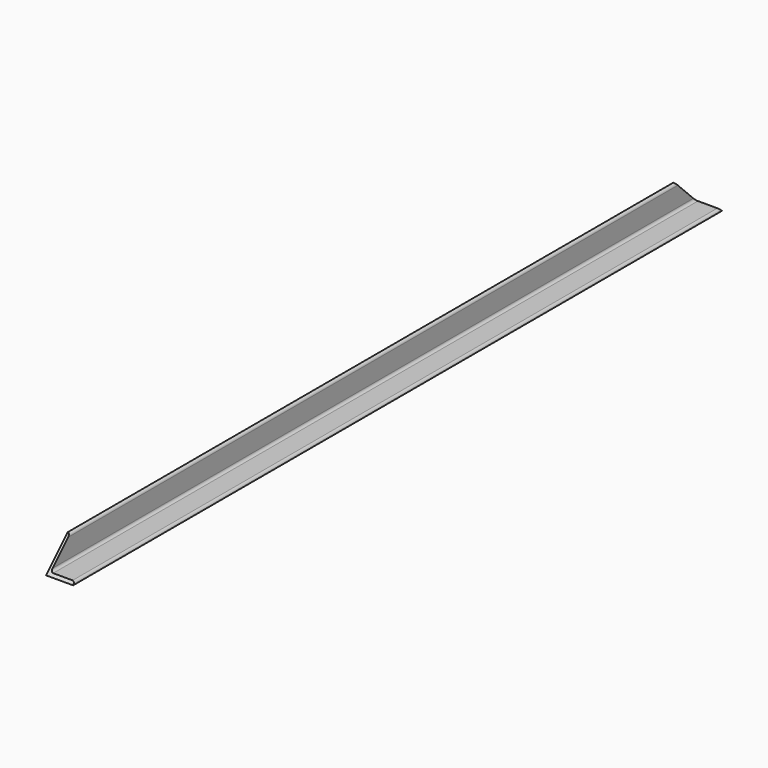
from build123d import *

# Parameters (mm, degrees)
F2_DEPTH = 1524
F4_DEPTH = 50.8


# Not quite as in the source:
# - a variable given as a bare number and used for a length is read in inches; the dataset says mm whatever the document's units were


with BuildPart() as f2:
    # F1 (on Front) → F2 (new body)
    with BuildSketch(Plane.XZ):
        with BuildLine():
            ThreePointArc((4.7625, -4.7625), (3.3675960454, -1.3949039546), (0, 0))
            Line((0, 0), (0, -50.8))
            Line((0, -50.8), (50.8, -50.8))
            ThreePointArc((50.8, -50.8), (49.4050960454, -47.4324039546), (46.0375, -46.0375))
            Line((46.0375, -46.0375), (9.525, -46.0375))
            ThreePointArc((9.525, -46.0375), (6.1574039546, -44.6425960454), (4.7625, -41.275))
            Line((4.7625, -41.275), (4.7625, -4.7625))
        make_face()
    extrude(amount=-F2_DEPTH)

    # F3 (on face) → F4 (cut)
    with BuildSketch(Plane(origin=(0, 0, 0), x_dir=(0, -1, 0), z_dir=(-1, 0, 0))):
        Polygon((-50.8, 0), (0, -50.8), (0, 0), align=None)
        Polygon((-1524, 0), (-1524, -50.8), (-1473.2, 0), align=None)
    extrude(amount=-F4_DEPTH, mode=Mode.SUBTRACT)


solid = f2.part
